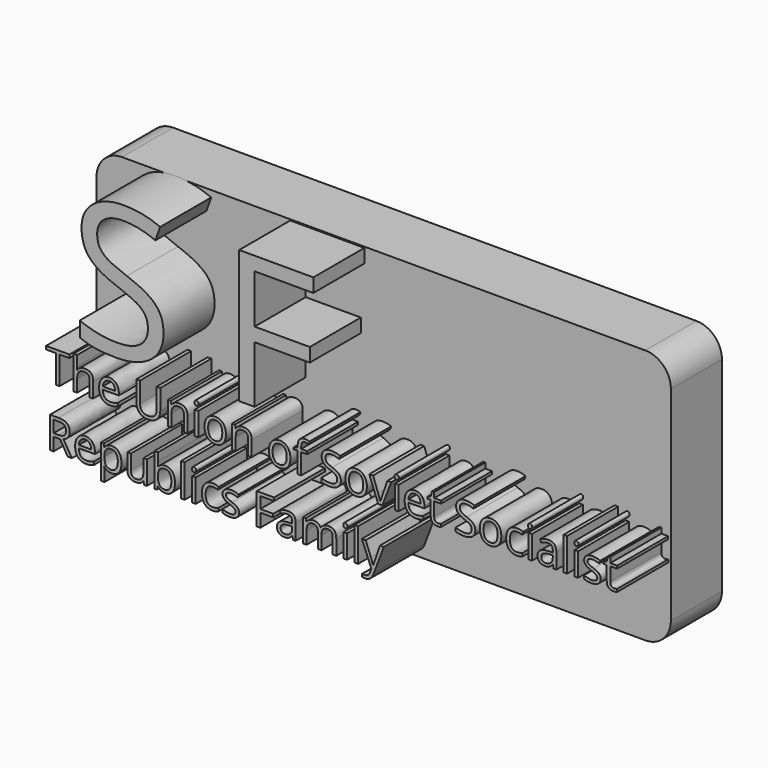
from build123d import *

# Parameters (mm, degrees)
F0_W         = 45
F0_H         = 20
F1_DEPTH     = 5
F2_TEXT_SIZE = 14.6018708647
F3_DEPTH     = 5
F4_TEXT_SIZE = 3.4189657629
F5_DEPTH     = 5
F6_R         = 2


# Not quite as in the source:
# - Text() gives the source's letters only with a copy of the font that has no kerning and outlines rounded to 1/6400 em; it was checked with that copy


with BuildPart() as f1:
    # F0 (on Front) → F1 (new body)
    with BuildSketch(Plane.XZ):
        with Locations((22.5, 10)):
            Rectangle(F0_W, F0_H)
    extrude(amount=F1_DEPTH)

    # F2 (on face) → F3 (join)
    with BuildSketch(Plane.XZ.offset(5)):
        with Locations((1.9339966, 9.4866529774)):
            Text('S F', F2_TEXT_SIZE, font='Open Sans', text_align=(TextAlign.LEFT, TextAlign.BOTTOM))
    extrude(amount=F3_DEPTH)

    # F4 (on face) → F5 (join)
    with BuildSketch(Plane.XZ.offset(5)):
        with Locations((0.0174870547, 5.9383441694)):
            Text('The Union of Soviet Socialist', F4_TEXT_SIZE, font='Open Sans', text_align=(TextAlign.LEFT, TextAlign.BOTTOM))
        with Locations((0.0174870547, 1.2885507319)):
            Text('Republics Family', F4_TEXT_SIZE, font='Open Sans', text_align=(TextAlign.LEFT, TextAlign.BOTTOM))
    extrude(amount=F5_DEPTH)

    # F6
    f6_edges = [f1.edges().sort_by_distance(p)[0] for p in [
        (0, -2.5, 20),
        (45, -2.5, 20),
        (45, -2.5, 0),
        (0, -2.5, 0),
    ]]
    fillet(f6_edges, radius=F6_R)


solid = f1.part
